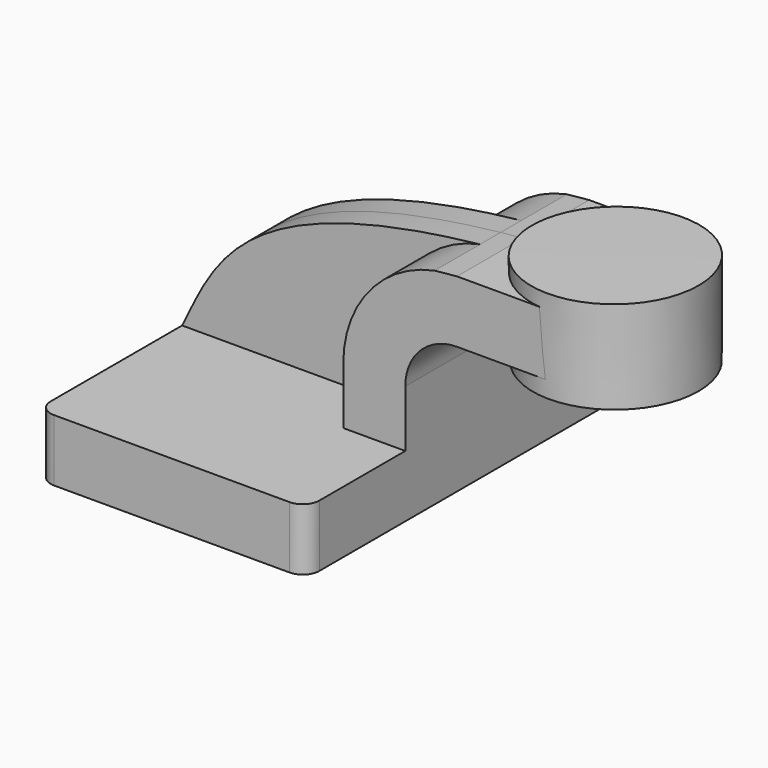
from build123d import *

# Parameters (mm, degrees)
F1_DEPTH  = 63.5
F2_DEPTH  = 25.4
F4_E5_0_W = 28.3572662234
F4_E5_0_H = 50.8
F5_DEPTH  = 19.05
F6_DEPTH  = 7.9375
F7_R      = 5.08


with BuildPart() as f1:
    # F0 (on Front) → F1 (new body, symmetric)
    with BuildSketch(Plane.XZ):
        Polygon((-41.275, 9.525), (-41.275, -9.525), (41.275, -9.525), (41.275, 9.525), (22.225, 9.525), align=None)
    extrude(amount=F1_DEPTH, both=True)

    # F0 (on Front) → F2 (join, symmetric)
    with BuildSketch(Plane.XZ):
        with BuildLine():
            Line((22.225, 9.525), (41.275, 9.525))
            Line((41.275, 9.525), (41.275, 27.0002))
            ThreePointArc((41.275, 27.0002), (45.9246798487, 38.2255201513), (57.15, 42.8752))
            Line((57.15, 42.8752), (60.325, 42.8752))
            Line((60.325, 42.8752), (60.325, 61.9252))
            Line((60.325, 61.9252), (57.15, 61.9252))
            add(Edge.make_bspline(
                [(50.2742596594, 61.2416926627), (52.505084267, 61.4836028987), (54.7963675205, 61.7116076427), (57.15, 61.9252)],
                knots=[108.25411783, 108.25411783, 108.25411783, 108.25411783, 111.5045361635, 111.5045361635, 111.5045361635, 111.5045361635], degree=3))
            ThreePointArc((50.2742596594, 61.2416926627), (30.1324977432, 49.1318559887), (22.225, 27.0002))
            Line((22.225, 27.0002), (22.225, 9.525))
        make_face()
    extrude(amount=F2_DEPTH, both=True)

    # F0 (on Front) → F3 (revolve)
    with BuildSketch(Plane.XZ):
        Polygon((85.5072662234, 66.675), (85.6886142667, 42.8752), (85.725, 38.1), (111.125, 38.1), (111.125, 66.675), align=None)
    revolve(axis=Axis((85.6161331117, 0, 52.3875), (-0.0076195085, 0, 0.9999709711)))

    # F4_E5_0 (on explicit) → F5 (join)
    with BuildSketch(Plane(origin=(57.15, 25.4, 61.9252), x_dir=(1, 0, 0), z_dir=(0, 0, -1))):
        with Locations((14.1786331117, 25.4)):
            Rectangle(F4_E5_0_W, F4_E5_0_H)
    extrude(amount=F5_DEPTH)

    # F0 (on Front) → F6 (join, symmetric)
    with BuildSketch(Plane.XZ):
        with BuildLine():
            add(Edge.make_bspline(
                [(-41.275, 9.525), (-31.2587030045, 29.7042218625), (-24.022623126, 53.1849514965), (50.2742596594, 61.2416926627)],
                knots=[0, 0, 0, 0, 108.25411783, 108.25411783, 108.25411783, 108.25411783], degree=3))
            Line((-41.275, 9.525), (22.225, 9.525))
            Line((22.225, 9.525), (22.225, 27.0002))
            ThreePointArc((22.225, 27.0002), (30.1324977432, 49.1318559887), (50.2742596594, 61.2416926627))
        make_face()
    extrude(amount=F6_DEPTH, both=True)

    # F7
    f7_edges = [f1.edges().sort_by_distance(p)[0] for p in [
        (41.275, -63.5, 0),
        (-41.275, -63.5, 0),
        (-41.275, 63.5, 0),
        (41.275, 63.5, 0),
    ]]
    fillet(f7_edges, radius=F7_R)


solid = f1.part
